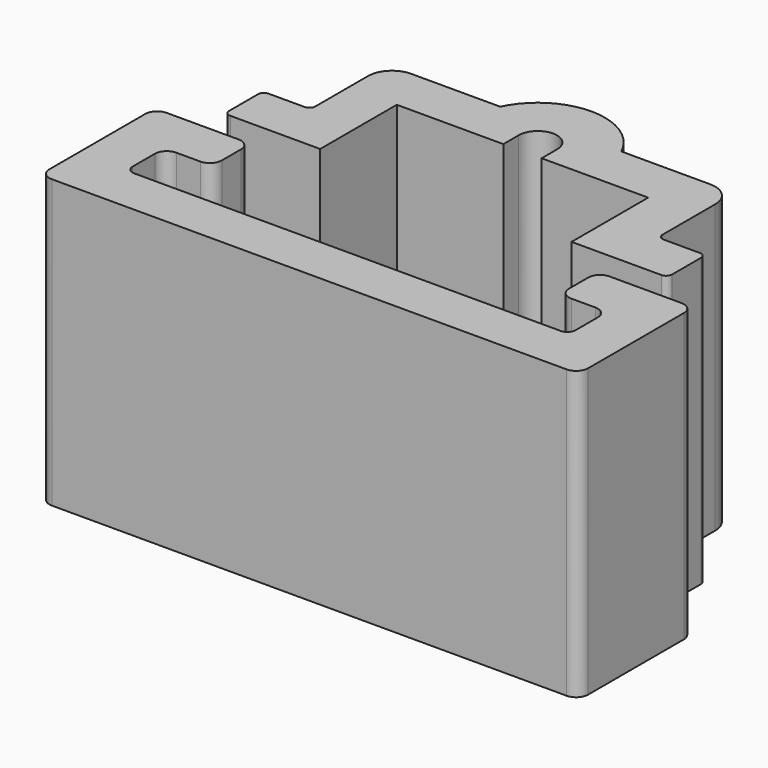
from build123d import *

# Parameters (mm, degrees)
F1_DEPTH = 6
F2_R     = 1
F3_R     = 0.25
F4_R     = 0.5
F5_R     = 0.35


# Not quite as in the source:
# - a feature names something its author has since deleted; it is built from what else it names


with BuildPart() as f1:
    # F0 (on Top) → F1 (new body, symmetric)
    with BuildSketch(Plane.XY):
        with BuildLine():
            Line((-9.0073623574, 2.6911826732), (-9.0073623574, 6.6911826732))
            Line((-9.0073623574, 6.6911826732), (-4.5573623574, 6.6911826732))
            Line((-4.5573623574, 6.6911826732), (-4.5573623574, 7.4911826732))
            ThreePointArc((-4.5573623574, 7.4911826732), (-4.3230477824, 8.0568680982), (-3.7573623574, 8.2911826732))
            ThreePointArc((-3.7573623574, 8.2911826732), (-3.1916769325, 8.0568680982), (-2.9573623574, 7.4911826732))
            Line((-2.9573623574, 7.4911826732), (-2.9573623574, 6.6911826732))
            Line((-2.9573623574, 6.6911826732), (1.4926376426, 6.6911826732))
            Line((1.4926376426, 6.6911826732), (1.4926376426, 2.6911826732))
            Line((1.4926376426, 2.6911826732), (3.4926376426, 2.6911826732))
            Line((3.4926376426, 2.6911826732), (5.4926376426, 2.6911826732))
            Line((5.4926376426, 2.6911826732), (5.4926376426, 4.6911826732))
            Line((5.4926376426, 4.6911826732), (3.4926376426, 4.6911826732))
            Line((3.4926376426, 4.6911826732), (3.4926376426, 8.6911826732))
            Line((3.4926376426, 8.6911826732), (-1.2275402293, 8.6911826732))
            ThreePointArc((-1.2275402293, 8.6911826732), (-2.2606994027, 9.8576145865), (-3.7573623574, 10.2911826732))
            ThreePointArc((-3.7573623574, 10.2911826732), (-5.2540253122, 9.8576145865), (-6.2871844856, 8.6911826732))
            Line((-6.2871844856, 8.6911826732), (-11.0073623574, 8.6911826732))
            Line((-11.0073623574, 8.6911826732), (-11.0073623574, 4.6911826732))
            Line((-11.0073623574, 4.6911826732), (-13.0073623574, 4.6911826732))
            Line((-13.0073623574, 4.6911826732), (-13.0073623574, 2.6911826732))
            Line((-13.0073623574, 2.6911826732), (-11.0073623574, 2.6911826732))
            Line((-11.0073623574, 2.6911826732), (-9.0073623574, 2.6911826732))
        make_face()
    extrude(amount=F1_DEPTH, both=True)

    # F2
    f2_edges = [f1.edges().sort_by_distance(p)[0] for p in [
        (-11.007362, 8.691183, 0),
        (3.492638, 8.691183, 0),
    ]]
    fillet(f2_edges, radius=F2_R)

    # F3
    f3_edges = [f1.edges().sort_by_distance(p)[0] for p in [
        (-11.007362, 4.691183, 0),
        (-13.007362, 4.691183, 0),
        (-13.007362, 2.691183, 0),
        (3.492638, 4.691183, 0),
        (5.492638, 4.691183, 0),
        (5.492638, 2.691183, 0),
    ]]
    fillet(f3_edges, radius=F3_R)


with BuildPart() as f1b:
    # F0 (on Top) → F1, piece 2 (new body, symmetric)
    with BuildSketch(Plane.XY):
        Polygon((5.4926376426, -2.4439409186), (-3.7573623574, -2.4439409186), (-13.0073623574, -2.4439409186), (-13.0073623574, -0.4439409186), (-11.0073623574, -0.4439409186), (-11.0073623574, 1.5560590814), (-15.0073623574, 1.5560590814), (-15.0073623574, -4.4439409186), (-3.7573623574, -4.4439409186), (7.4926376426, -4.4439409186), (7.4926376426, 1.5560590814), (3.4926376426, 1.5560590814), (3.4926376426, -0.4439409186), (5.4926376426, -0.4439409186), align=None)
    extrude(amount=F1_DEPTH, both=True)

    # F4
    f4_edges = [f1b.edges().sort_by_distance(p)[0] for p in [
        (3.492638, -0.443941, 0),
        (5.492638, -0.443941, 0),
        (-11.007362, 1.556059, 0),
        (3.492638, 1.556059, 0),
        (-15.007362, 1.556059, 0),
        (7.492638, 1.556059, 0),
        (-15.007362, -4.443941, 0),
        (7.492638, -4.443941, 0),
        (-11.007362, -0.443941, 0),
        (-13.007362, -0.443941, 0),
    ]]
    fillet(f4_edges, radius=F4_R)

    # F5
    f5_edges = [f1b.edges().sort_by_distance(p)[0] for p in [
        (-13.007362, -2.443941, 0),
        (5.492638, -2.443941, 0),
    ]]
    fillet(f5_edges, radius=F5_R)


solid = Compound([f1.part, f1b.part])
